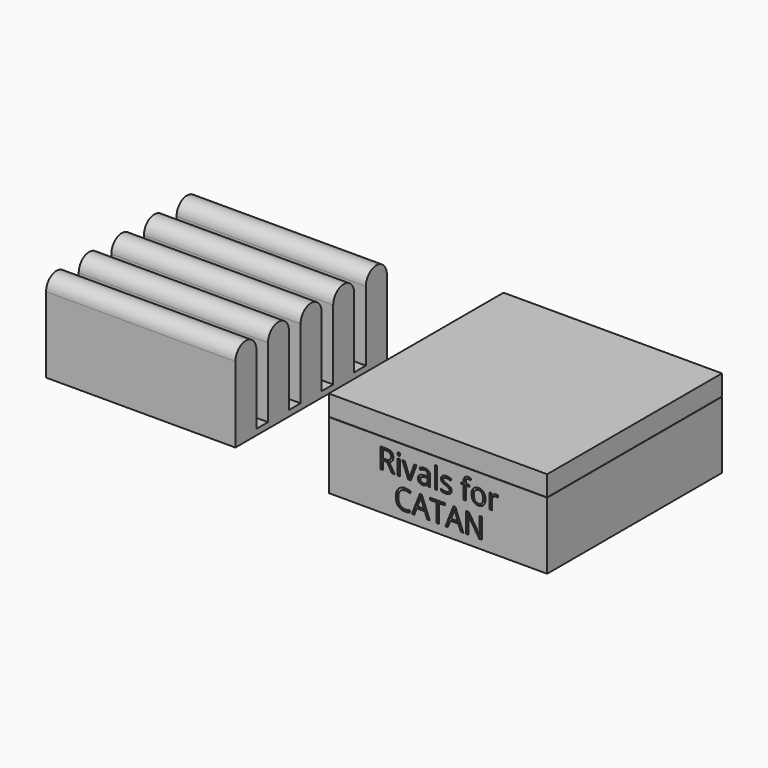
from build123d import *

# Parameters (mm, degrees)
F0_W          = 75
F0_H          = 75
F1_DEPTH      = 2
F0_W_2        = 65
F0_H_2        = 65
F2_W          = 75
F2_H          = 75
F2_W_2        = 71
F2_H_2        = 71
F3_DEPTH      = 26
F4_W          = 75
F4_H          = 75
F4_W_2        = 72.4
F4_H_2        = 72.4
F5_DEPTH      = 5
F7_W          = 75
F7_H          = 75
F8_DEPTH      = 2
F9_W          = 75
F9_H          = 75
F9_W_2        = 73.6
F9_H_2        = 73.6
F10_DEPTH     = 5
F11_TEXT_SIZE = 9.7222222222
F12_DEPTH     = 0.5
F14_DEPTH     = 65


# Not quite as in the source:
# - Text() gives the source's letters only with a copy of the font that has no kerning and outlines rounded to 1/6400 em; it was checked with that copy


with BuildPart() as f1:
    # F0 (on Top) → F1 (new body)
    with BuildSketch(Plane.XY):
        Rectangle(F0_W, F0_H)
    extrude(amount=F1_DEPTH)

    # F2 (on face) → F3 (join)
    with BuildSketch(Plane.XY.offset(2)):
        Rectangle(F2_W, F2_H)
        Rectangle(F2_W_2, F2_H_2, mode=Mode.SUBTRACT)
    extrude(amount=F3_DEPTH)

    # F4 (on face) → F5 (cut)
    with BuildSketch(Plane.XY.offset(28)):
        Rectangle(F4_W, F4_H)
        Rectangle(F4_W_2, F4_H_2, mode=Mode.SUBTRACT)
    extrude(amount=-F5_DEPTH, mode=Mode.SUBTRACT)

    # F11 (on face) → F12 (cut)
    with BuildSketch(Plane.XZ.offset(37.5)):
        with Locations((-20.6840277778, 13)):
            Text('Rivals for', F11_TEXT_SIZE, font='Open Sans', text_align=(TextAlign.LEFT, TextAlign.BOTTOM))
        with Locations((-15.0967881944, 3)):
            Text('CATAN', F11_TEXT_SIZE, font='Open Sans', text_align=(TextAlign.LEFT, TextAlign.BOTTOM))
    extrude(amount=-F12_DEPTH, mode=Mode.SUBTRACT)


with BuildPart() as f1b:
    # F0 (on Top) → F1, piece 2 (new body)
    with BuildSketch(Plane.XY):
        with Locations((-106.066017178, 0)):
            Rectangle(F0_W_2, F0_H_2)
    extrude(amount=F1_DEPTH)

    # F13 (on face) → F14 (join)
    with BuildSketch(Plane.YZ.offset(-73.566017178)):
        with BuildLine():
            Line((-32.5, 26), (-32.5, 2))
            Line((-32.5, 2), (-23.5, 2))
            Line((-23.5, 2), (-23.5, 26))
            ThreePointArc((-23.5, 26), (-28, 30.5), (-32.5, 26))
        make_face()
        with BuildLine():
            Line((-18.5, 26), (-18.5, 2))
            Line((-18.5, 2), (-9.5, 2))
            Line((-9.5, 2), (-9.5, 26))
            ThreePointArc((-9.5, 26), (-14, 30.5), (-18.5, 26))
        make_face()
        with BuildLine():
            Line((-4.5, 26), (-4.5, 2))
            Line((-4.5, 2), (4.5, 2))
            Line((4.5, 2), (4.5, 26))
            ThreePointArc((4.5, 26), (0, 30.5), (-4.5, 26))
        make_face()
        with BuildLine():
            Line((9.5, 2), (18.5, 2))
            Line((18.5, 2), (18.5, 26))
            ThreePointArc((18.5, 26), (14, 30.5), (9.5, 26))
            Line((9.5, 26), (9.5, 2))
        make_face()
        with BuildLine():
            Line((23.5, 2), (32.5, 2))
            Line((32.5, 2), (32.5, 26))
            ThreePointArc((32.5, 26), (28, 30.5), (23.5, 26))
            Line((23.5, 26), (23.5, 2))
        make_face()
    extrude(amount=-F14_DEPTH)


with BuildPart() as f8:
    # F7 (on offset) → F8 (new body)
    with BuildSketch(Plane.XY.offset(28.1)):
        Rectangle(F7_W, F7_H)
    extrude(amount=F8_DEPTH)

    # F9 (on face) → F10 (join)
    with BuildSketch(Plane(origin=(0, 0, 28.1), x_dir=(1, 0, 0), z_dir=(0, 0, -1))):
        Rectangle(F9_W, F9_H)
        Rectangle(F9_W_2, F9_H_2, mode=Mode.SUBTRACT)
    extrude(amount=F10_DEPTH)


solid = Compound([f1.part, f1b.part, f8.part])
